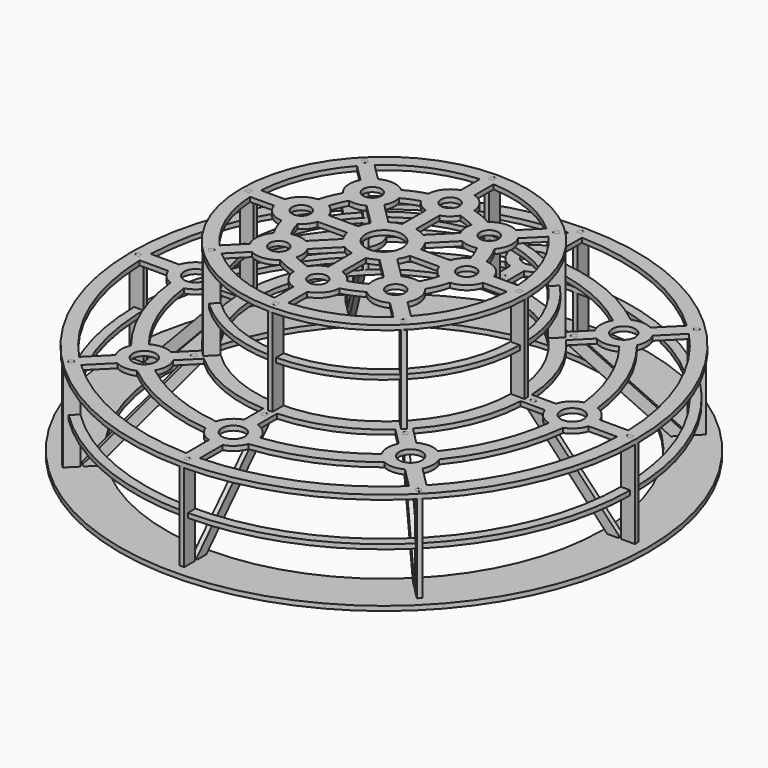
from build123d import *

# Parameters (mm, degrees)
F4_R      = 550
F4_R_2    = 25
F4_R_3    = 280
F5_DEPTH  = 10
F6_R      = 310
F6_R_2    = 20
F6_R_3    = 40
F7_DEPTH  = 10
F8_R      = 575
F8_R_2    = 475
F9_DEPTH  = 10
F11_DEPTH = 5
F12_COUNT = 8
F13_R     = 520
F14_DEPTH = 10
F15_R     = 280
F16_DEPTH = 10
F17_COUNT = 8


with BuildPart() as f5:
    # F4 (on Top) → F5 (new body)
    with BuildSketch(Plane.XY):
        Circle(F4_R)
        Polygon((-374.0594872477, -375.4737008101), (-371.3017708011, -378.2314172567), (-378.3728386129, -385.3024850685), (-381.1305550595, -382.5447686219), (-382.5447686219, -382.5447686219), (-382.5447686219, -381.1305550595), (-385.3024850685, -378.3728386129), (-378.2314172567, -371.3017708011), (-375.4737008101, -374.0594872477), (-374.0594872477, -374.0594872477), align=None, mode=Mode.SUBTRACT)
        with Locations((-289.9137802865, -289.9137802865)):
            Circle(F4_R_2, mode=Mode.SUBTRACT)
        with BuildLine():
            ThreePointArc((-46.8602222393, -427.4390243902), (-34.4319247471, -446.2552418033), (-15, -457.6969600708))
            Line((-15, -457.6969600708), (-15, -519.783608822))
            ThreePointArc((-15, -519.783608822), (-198.9953848298, -480.4173569059), (-356.9359128298, -378.1491162654))
            Line((-356.9359128298, -378.1491162654), (-313.0340224768, -334.2472259124))
            ThreePointArc((-313.0340224768, -334.2472259124), (-291.2030601412, -339.8971550971), (-269.1098517768, -335.3802136034))
            ThreePointArc((-269.1098517768, -335.3802136034), (-164.553875917, -397.2681989799), (-46.8602222393, -427.4390243902))
        make_face(mode=Mode.SUBTRACT)
        with BuildLine():
            Line((-15, -309.6368841078), (-15, -362.3030399292))
            ThreePointArc((-15, -362.3030399292), (-36.1104599854, -375.4162656782), (-48.3000733443, -397.0731707317))
            ThreePointArc((-48.3000733443, -397.0731707317), (-153.073372946, -369.5518130045), (-246.619822258, -314.9264410452))
            ThreePointArc((-246.619822258, -314.9264410452), (-239.9254361013, -290.9933383562), (-245.5803346606, -266.7935380962))
            Line((-245.5803346606, -266.7935380962), (-208.3397387403, -229.5529421759))
            ThreePointArc((-208.3397387403, -229.5529421759), (-118.6318640332, -286.4026550785), (-15, -309.6368841078))
        make_face(mode=Mode.SUBTRACT)
        with BuildLine():
            Line((-519.783608822, -15), (-457.6969600708, -15))
            ThreePointArc((-457.6969600708, -15), (-446.2552418033, -34.4319247471), (-427.4390243902, -46.8602222393))
            ThreePointArc((-427.4390243902, -46.8602222393), (-397.2681989799, -164.553875917), (-335.3802136034, -269.1098517768))
            ThreePointArc((-335.3802136034, -269.1098517768), (-339.8971550971, -291.2030601412), (-334.2472259124, -313.0340224768))
            Line((-334.2472259124, -313.0340224768), (-378.1491162654, -356.9359128298))
            ThreePointArc((-378.1491162654, -356.9359128298), (-480.4173569059, -198.9953848298), (-519.783608822, -15))
        make_face(mode=Mode.SUBTRACT)
        with BuildLine():
            ThreePointArc((-397.0731707317, -48.3000733443), (-375.4162656782, -36.1104599854), (-362.3030399292, -15))
            Line((-362.3030399292, -15), (-309.6368841078, -15))
            ThreePointArc((-309.6368841078, -15), (-286.4026550785, -118.6318640332), (-229.5529421759, -208.3397387403))
            Line((-229.5529421759, -208.3397387403), (-266.7935380962, -245.5803346606))
            ThreePointArc((-266.7935380962, -245.5803346606), (-290.9933383562, -239.9254361013), (-314.9264410452, -246.619822258))
            ThreePointArc((-314.9264410452, -246.619822258), (-369.5518130045, -153.073372946), (-397.0731707317, -48.3000733443))
        make_face(mode=Mode.SUBTRACT)
        Polygon((-236.8100610194, -229.8804145637), (-229.7389932075, -222.8093467519), (-226.9812767609, -225.5670631985), (-225.5670631985, -225.5670631985), (-225.5670631985, -226.9812767609), (-222.8093467519, -229.7389932075), (-229.8804145637, -236.8100610194), (-232.6381310104, -234.0523445727), (-234.0523445727, -234.0523445727), (-234.0523445727, -232.6381310104), align=None, mode=Mode.SUBTRACT)
        Polygon((-215.5968575838, -208.6672111282), (-208.5257897719, -201.5961433163), (-205.7680733253, -204.3538597629), (-204.3538597629, -204.3538597629), (-204.3538597629, -205.7680733253), (-201.5961433163, -208.5257897719), (-208.6672111282, -215.5968575838), (-211.4249275748, -212.8391411372), (-212.8391411372, -212.8391411372), (-212.8391411372, -211.4249275748), align=None, mode=Mode.SUBTRACT)
        Polygon((1, -530), (4.9, -530), (4.9, -540), (1, -540), (0, -541), (-1, -540), (-4.9, -540), (-4.9, -530), (-1, -530), (0, -529), align=None, mode=Mode.SUBTRACT)
        with BuildLine():
            ThreePointArc((356.9359128298, -378.1491162654), (198.9953848298, -480.4173569059), (15, -519.783608822))
            Line((15, -519.783608822), (15, -457.6969600708))
            ThreePointArc((15, -457.6969600708), (34.4319247471, -446.2552418033), (46.8602222393, -427.4390243902))
            ThreePointArc((46.8602222393, -427.4390243902), (164.553875917, -397.2681989799), (269.1098517768, -335.3802136034))
            ThreePointArc((269.1098517768, -335.3802136034), (291.2030601412, -339.8971550971), (313.0340224768, -334.2472259124))
            Line((313.0340224768, -334.2472259124), (356.9359128298, -378.1491162654))
        make_face(mode=Mode.SUBTRACT)
        with Locations((0, -410)):
            Circle(F4_R_2, mode=Mode.SUBTRACT)
        Polygon((-4.9, -330), (-4.9, -320), (-1, -320), (0, -319), (1, -320), (4.9, -320), (4.9, -330), (1, -330), (0, -331), (-1, -330), align=None, mode=Mode.SUBTRACT)
        Polygon((-4.9, -300), (-4.9, -290), (-1, -290), (0, -289), (1, -290), (4.9, -290), (4.9, -300), (1, -300), (0, -301), (-1, -300), align=None, mode=Mode.SUBTRACT)
        with BuildLine():
            ThreePointArc((246.619822258, -314.9264410452), (153.073372946, -369.5518130045), (48.3000733443, -397.0731707317))
            ThreePointArc((48.3000733443, -397.0731707317), (36.1104599854, -375.4162656782), (15, -362.3030399292))
            Line((15, -362.3030399292), (15, -309.6368841078))
            ThreePointArc((15, -309.6368841078), (118.6318640332, -286.4026550785), (208.3397387403, -229.5529421759))
            Line((208.3397387403, -229.5529421759), (245.5803346606, -266.7935380962))
            ThreePointArc((245.5803346606, -266.7935380962), (239.9254361013, -290.9933383562), (246.619822258, -314.9264410452))
        make_face(mode=Mode.SUBTRACT)
        Polygon((375.4737008101, -374.0594872477), (378.2314172567, -371.3017708011), (385.3024850685, -378.3728386129), (382.5447686219, -381.1305550595), (382.5447686219, -382.5447686219), (381.1305550595, -382.5447686219), (378.3728386129, -385.3024850685), (371.3017708011, -378.2314172567), (374.0594872477, -375.4737008101), (374.0594872477, -374.0594872477), align=None, mode=Mode.SUBTRACT)
        with Locations((289.9137802865, -289.9137802865)):
            Circle(F4_R_2, mode=Mode.SUBTRACT)
        Polygon((229.8804145637, -236.8100610194), (222.8093467519, -229.7389932075), (225.5670631985, -226.9812767609), (225.5670631985, -225.5670631985), (226.9812767609, -225.5670631985), (229.7389932075, -222.8093467519), (236.8100610194, -229.8804145637), (234.0523445727, -232.6381310104), (234.0523445727, -234.0523445727), (232.6381310104, -234.0523445727), align=None, mode=Mode.SUBTRACT)
        Polygon((208.6672111282, -215.5968575838), (201.5961433163, -208.5257897719), (204.3538597629, -205.7680733253), (204.3538597629, -204.3538597629), (205.7680733253, -204.3538597629), (208.5257897719, -201.5961433163), (215.5968575838, -208.6672111282), (212.8391411372, -211.4249275748), (212.8391411372, -212.8391411372), (211.4249275748, -212.8391411372), align=None, mode=Mode.SUBTRACT)
        with BuildLine():
            Line((378.1491162654, -356.9359128298), (334.2472259124, -313.0340224768))
            ThreePointArc((334.2472259124, -313.0340224768), (339.8971550971, -291.2030601412), (335.3802136034, -269.1098517768))
            ThreePointArc((335.3802136034, -269.1098517768), (397.2681989799, -164.553875917), (427.4390243902, -46.8602222393))
            ThreePointArc((427.4390243902, -46.8602222393), (446.2552418033, -34.4319247471), (457.6969600708, -15))
            Line((457.6969600708, -15), (519.783608822, -15))
            ThreePointArc((519.783608822, -15), (480.4173569059, -198.9953848298), (378.1491162654, -356.9359128298))
        make_face(mode=Mode.SUBTRACT)
        with BuildLine():
            ThreePointArc((314.9264410452, -246.619822258), (290.9933383562, -239.9254361013), (266.7935380962, -245.5803346606))
            Line((266.7935380962, -245.5803346606), (229.5529421759, -208.3397387403))
            ThreePointArc((229.5529421759, -208.3397387403), (286.4026550785, -118.6318640332), (309.6368841078, -15))
            Line((309.6368841078, -15), (362.3030399292, -15))
            ThreePointArc((362.3030399292, -15), (375.4162656782, -36.1104599854), (397.0731707317, -48.3000733443))
            ThreePointArc((397.0731707317, -48.3000733443), (369.5518130045, -153.073372946), (314.9264410452, -246.619822258))
        make_face(mode=Mode.SUBTRACT)
        Polygon((-530, -1), (-530, -4.9), (-540, -4.9), (-540, -1), (-541, 0), (-540, 1), (-540, 4.9), (-530, 4.9), (-530, 1), (-529, 0), align=None, mode=Mode.SUBTRACT)
        with Locations((-410, 0)):
            Circle(F4_R_2, mode=Mode.SUBTRACT)
        Polygon((-330, 4.9), (-320, 4.9), (-320, 1), (-319, 0), (-320, -1), (-320, -4.9), (-330, -4.9), (-330, -1), (-331, 0), (-330, 1), align=None, mode=Mode.SUBTRACT)
        Polygon((-300, 4.9), (-290, 4.9), (-290, 1), (-289, 0), (-290, -1), (-290, -4.9), (-300, -4.9), (-300, -1), (-301, 0), (-300, 1), align=None, mode=Mode.SUBTRACT)
        with BuildLine():
            ThreePointArc((-314.9264410452, 246.619822258), (-290.9933383562, 239.9254361013), (-266.7935380962, 245.5803346606))
            Line((-266.7935380962, 245.5803346606), (-229.5529421759, 208.3397387403))
            ThreePointArc((-229.5529421759, 208.3397387403), (-286.4026550785, 118.6318640332), (-309.6368841078, 15))
            Line((-309.6368841078, 15), (-362.3030399292, 15))
            ThreePointArc((-362.3030399292, 15), (-375.4162656782, 36.1104599854), (-397.0731707317, 48.3000733443))
            ThreePointArc((-397.0731707317, 48.3000733443), (-369.5518130045, 153.073372946), (-314.9264410452, 246.619822258))
        make_face(mode=Mode.SUBTRACT)
        with BuildLine():
            Line((-378.1491162654, 356.9359128298), (-334.2472259124, 313.0340224768))
            ThreePointArc((-334.2472259124, 313.0340224768), (-339.8971550971, 291.2030601412), (-335.3802136034, 269.1098517768))
            ThreePointArc((-335.3802136034, 269.1098517768), (-397.2681989799, 164.553875917), (-427.4390243902, 46.8602222393))
            ThreePointArc((-427.4390243902, 46.8602222393), (-446.2552418033, 34.4319247471), (-457.6969600708, 15))
            Line((-457.6969600708, 15), (-519.783608822, 15))
            ThreePointArc((-519.783608822, 15), (-480.4173569059, 198.9953848298), (-378.1491162654, 356.9359128298))
        make_face(mode=Mode.SUBTRACT)
        Polygon((-208.6672111282, 215.5968575838), (-201.5961433163, 208.5257897719), (-204.3538597629, 205.7680733253), (-204.3538597629, 204.3538597629), (-205.7680733253, 204.3538597629), (-208.5257897719, 201.5961433163), (-215.5968575838, 208.6672111282), (-212.8391411372, 211.4249275748), (-212.8391411372, 212.8391411372), (-211.4249275748, 212.8391411372), align=None, mode=Mode.SUBTRACT)
        Polygon((-229.8804145637, 236.8100610194), (-222.8093467519, 229.7389932075), (-225.5670631985, 226.9812767609), (-225.5670631985, 225.5670631985), (-226.9812767609, 225.5670631985), (-229.7389932075, 222.8093467519), (-236.8100610194, 229.8804145637), (-234.0523445727, 232.6381310104), (-234.0523445727, 234.0523445727), (-232.6381310104, 234.0523445727), align=None, mode=Mode.SUBTRACT)
        with Locations((-289.9137802865, 289.9137802865)):
            Circle(F4_R_2, mode=Mode.SUBTRACT)
        Polygon((-375.4737008101, 374.0594872477), (-378.2314172567, 371.3017708011), (-385.3024850685, 378.3728386129), (-382.5447686219, 381.1305550595), (-382.5447686219, 382.5447686219), (-381.1305550595, 382.5447686219), (-378.3728386129, 385.3024850685), (-371.3017708011, 378.2314172567), (-374.0594872477, 375.4737008101), (-374.0594872477, 374.0594872477), align=None, mode=Mode.SUBTRACT)
        with BuildLine():
            ThreePointArc((-48.3000733443, 397.0731707317), (-36.1104599854, 375.4162656782), (-15, 362.3030399292))
            Line((-15, 362.3030399292), (-15, 309.6368841078))
            ThreePointArc((-15, 309.6368841078), (-118.6318640332, 286.4026550785), (-208.3397387403, 229.5529421759))
            Line((-208.3397387403, 229.5529421759), (-245.5803346606, 266.7935380962))
            ThreePointArc((-245.5803346606, 266.7935380962), (-239.9254361013, 290.9933383562), (-246.619822258, 314.9264410452))
            ThreePointArc((-246.619822258, 314.9264410452), (-153.073372946, 369.5518130045), (-48.3000733443, 397.0731707317))
        make_face(mode=Mode.SUBTRACT)
        with BuildLine():
            Line((-15, 519.783608822), (-15, 457.6969600708))
            ThreePointArc((-15, 457.6969600708), (-34.4319247471, 446.2552418033), (-46.8602222393, 427.4390243902))
            ThreePointArc((-46.8602222393, 427.4390243902), (-164.553875917, 397.2681989799), (-269.1098517768, 335.3802136034))
            ThreePointArc((-269.1098517768, 335.3802136034), (-291.2030601412, 339.8971550971), (-313.0340224768, 334.2472259124))
            Line((-313.0340224768, 334.2472259124), (-356.9359128298, 378.1491162654))
            ThreePointArc((-356.9359128298, 378.1491162654), (-198.9953848298, 480.4173569059), (-15, 519.783608822))
        make_face(mode=Mode.SUBTRACT)
        Circle(F4_R_3, mode=Mode.SUBTRACT)
        Polygon((215.5968575838, 208.6672111282), (208.5257897719, 201.5961433163), (205.7680733253, 204.3538597629), (204.3538597629, 204.3538597629), (204.3538597629, 205.7680733253), (201.5961433163, 208.5257897719), (208.6672111282, 215.5968575838), (211.4249275748, 212.8391411372), (212.8391411372, 212.8391411372), (212.8391411372, 211.4249275748), align=None, mode=Mode.SUBTRACT)
        Polygon((236.8100610194, 229.8804145637), (229.7389932075, 222.8093467519), (226.9812767609, 225.5670631985), (225.5670631985, 225.5670631985), (225.5670631985, 226.9812767609), (222.8093467519, 229.7389932075), (229.8804145637, 236.8100610194), (232.6381310104, 234.0523445727), (234.0523445727, 234.0523445727), (234.0523445727, 232.6381310104), align=None, mode=Mode.SUBTRACT)
        Polygon((300, -4.9), (290, -4.9), (290, -1), (289, 0), (290, 1), (290, 4.9), (300, 4.9), (300, 1), (301, 0), (300, -1), align=None, mode=Mode.SUBTRACT)
        Polygon((330, -4.9), (320, -4.9), (320, -1), (319, 0), (320, 1), (320, 4.9), (330, 4.9), (330, 1), (331, 0), (330, -1), align=None, mode=Mode.SUBTRACT)
        with Locations((410, 0)):
            Circle(F4_R_2, mode=Mode.SUBTRACT)
        with BuildLine():
            ThreePointArc((397.0731707317, 48.3000733443), (375.4162656782, 36.1104599854), (362.3030399292, 15))
            Line((362.3030399292, 15), (309.6368841078, 15))
            ThreePointArc((309.6368841078, 15), (286.4026550785, 118.6318640332), (229.5529421759, 208.3397387403))
            Line((229.5529421759, 208.3397387403), (266.7935380962, 245.5803346606))
            ThreePointArc((266.7935380962, 245.5803346606), (290.9933383562, 239.9254361013), (314.9264410452, 246.619822258))
            ThreePointArc((314.9264410452, 246.619822258), (369.5518130045, 153.073372946), (397.0731707317, 48.3000733443))
        make_face(mode=Mode.SUBTRACT)
        Polygon((530, 1), (530, 4.9), (540, 4.9), (540, 1), (541, 0), (540, -1), (540, -4.9), (530, -4.9), (530, -1), (529, 0), align=None, mode=Mode.SUBTRACT)
        with BuildLine():
            Line((519.783608822, 15), (457.6969600708, 15))
            ThreePointArc((457.6969600708, 15), (446.2552418033, 34.4319247471), (427.4390243902, 46.8602222393))
            ThreePointArc((427.4390243902, 46.8602222393), (397.2681989799, 164.553875917), (335.3802136034, 269.1098517768))
            ThreePointArc((335.3802136034, 269.1098517768), (339.8971550971, 291.2030601412), (334.2472259124, 313.0340224768))
            Line((334.2472259124, 313.0340224768), (378.1491162654, 356.9359128298))
            ThreePointArc((378.1491162654, 356.9359128298), (480.4173569059, 198.9953848298), (519.783608822, 15))
        make_face(mode=Mode.SUBTRACT)
        Polygon((4.9, 300), (4.9, 290), (1, 290), (0, 289), (-1, 290), (-4.9, 290), (-4.9, 300), (-1, 300), (0, 301), (1, 300), align=None, mode=Mode.SUBTRACT)
        Polygon((4.9, 330), (4.9, 320), (1, 320), (0, 319), (-1, 320), (-4.9, 320), (-4.9, 330), (-1, 330), (0, 331), (1, 330), align=None, mode=Mode.SUBTRACT)
        with BuildLine():
            ThreePointArc((246.619822258, 314.9264410452), (239.9254361013, 290.9933383562), (245.5803346606, 266.7935380962))
            Line((245.5803346606, 266.7935380962), (208.3397387403, 229.5529421759))
            ThreePointArc((208.3397387403, 229.5529421759), (118.6318640332, 286.4026550785), (15, 309.6368841078))
            Line((15, 309.6368841078), (15, 362.3030399292))
            ThreePointArc((15, 362.3030399292), (36.1104599854, 375.4162656782), (48.3000733443, 397.0731707317))
            ThreePointArc((48.3000733443, 397.0731707317), (153.073372946, 369.5518130045), (246.619822258, 314.9264410452))
        make_face(mode=Mode.SUBTRACT)
        with Locations((0, 410)):
            Circle(F4_R_2, mode=Mode.SUBTRACT)
        Polygon((4.9, 540), (4.9, 530), (1, 530), (0, 529), (-1, 530), (-4.9, 530), (-4.9, 540), (-1, 540), (0, 541), (1, 540), align=None, mode=Mode.SUBTRACT)
        with BuildLine():
            Line((356.9359128298, 378.1491162654), (313.0340224768, 334.2472259124))
            ThreePointArc((313.0340224768, 334.2472259124), (291.2030601412, 339.8971550971), (269.1098517768, 335.3802136034))
            ThreePointArc((269.1098517768, 335.3802136034), (164.553875917, 397.2681989799), (46.8602222393, 427.4390243902))
            ThreePointArc((46.8602222393, 427.4390243902), (34.4319247471, 446.2552418033), (15, 457.6969600708))
            Line((15, 457.6969600708), (15, 519.783608822))
            ThreePointArc((15, 519.783608822), (198.9953848298, 480.4173569059), (356.9359128298, 378.1491162654))
        make_face(mode=Mode.SUBTRACT)
        with Locations((289.9137802865, 289.9137802865)):
            Circle(F4_R_2, mode=Mode.SUBTRACT)
        Polygon((374.0594872477, 375.4737008101), (371.3017708011, 378.2314172567), (378.3728386129, 385.3024850685), (381.1305550595, 382.5447686219), (382.5447686219, 382.5447686219), (382.5447686219, 381.1305550595), (385.3024850685, 378.3728386129), (378.2314172567, 371.3017708011), (375.4737008101, 374.0594872477), (374.0594872477, 374.0594872477), align=None, mode=Mode.SUBTRACT)
    extrude(amount=F5_DEPTH)


with BuildPart() as f7:
    # F6 (on offset) → F7 (new body)
    with BuildSketch(Plane.XY.offset(200)):
        Circle(F6_R)
        Polygon((-204.3538597629, -204.3538597629), (-204.3538597629, -205.7680733253), (-201.5961433163, -208.5257897719), (-208.6672111282, -215.5968575838), (-211.4249275748, -212.8391411372), (-212.8391411372, -212.8391411372), (-212.8391411372, -211.4249275748), (-215.5968575838, -208.6672111282), (-208.5257897719, -201.5961433163), (-205.7680733253, -204.3538597629), align=None, mode=Mode.SUBTRACT)
        with BuildLine():
            ThreePointArc((-49.888765157, -183.3333333333), (-39.3023002536, -210.9084000682), (-15, -227.6969600708))
            Line((-15, -227.6969600708), (-15, -279.5979256003))
            ThreePointArc((-15, -279.5979256003), (-107.1513610622, -258.6862691032), (-187.0989874799, -208.3121909155))
            Line((-187.0989874799, -208.3121909155), (-150.3994628039, -171.6126662395))
            ThreePointArc((-150.3994628039, -171.6126662395), (-121.3438368718, -176.925682923), (-94.35955907, -164.9129273651))
            ThreePointArc((-94.35955907, -164.9129273651), (-72.7098521494, -175.5371111771), (-49.888765157, -183.3333333333))
        make_face(mode=Mode.SUBTRACT)
        with BuildLine():
            Line((-279.5979256003, -15), (-227.6969600708, -15))
            ThreePointArc((-227.6969600708, -15), (-210.9084000682, -39.3023002536), (-183.3333333333, -49.888765157))
            ThreePointArc((-183.3333333333, -49.888765157), (-175.5371111771, -72.7098521494), (-164.9129273651, -94.35955907))
            ThreePointArc((-164.9129273651, -94.35955907), (-176.925682923, -121.3438368718), (-171.6126662395, -150.3994628039))
            Line((-171.6126662395, -150.3994628039), (-208.3121909155, -187.0989874799))
            ThreePointArc((-208.3121909155, -187.0989874799), (-258.6862691032, -107.1513610622), (-279.5979256003, -15))
        make_face(mode=Mode.SUBTRACT)
        with Locations((-127.2792206136, -127.2792206136)):
            Circle(F6_R_2, mode=Mode.SUBTRACT)
        with BuildLine():
            Line((-15, -68.3739716559), (-15, -132.3030399292))
            ThreePointArc((-15, -132.3030399292), (-30.9028195191, -140.6933116916), (-42.8093317968, -154.1666666667))
            ThreePointArc((-42.8093317968, -154.1666666667), (-61.2293491784, -147.8207252018), (-78.7415266213, -139.2830642445))
            ThreePointArc((-78.7415266213, -139.2830642445), (-77.633601525, -121.3367880044), (-82.9457749877, -104.1589784233))
            Line((-82.9457749877, -104.1589784233), (-37.7410972967, -58.9543007323))
            ThreePointArc((-37.7410972967, -58.9543007323), (-26.7878402656, -64.6715672758), (-15, -68.3739716559))
        make_face(mode=Mode.SUBTRACT)
        with BuildLine():
            Line((-132.3030399292, -15), (-68.3739716559, -15))
            ThreePointArc((-68.3739716559, -15), (-64.6715672758, -26.7878402656), (-58.9543007323, -37.7410972967))
            Line((-58.9543007323, -37.7410972967), (-104.1589784233, -82.9457749877))
            ThreePointArc((-104.1589784233, -82.9457749877), (-121.3367880044, -77.633601525), (-139.2830642445, -78.7415266213))
            ThreePointArc((-139.2830642445, -78.7415266213), (-147.8207252018, -61.2293491784), (-154.1666666667, -42.8093317968))
            ThreePointArc((-154.1666666667, -42.8093317968), (-140.6933116916, -30.9028195191), (-132.3030399292, -15))
        make_face(mode=Mode.SUBTRACT)
        Polygon((0, -289), (1, -290), (4.9, -290), (4.9, -300), (1, -300), (0, -301), (-1, -300), (-4.9, -300), (-4.9, -290), (-1, -290), align=None, mode=Mode.SUBTRACT)
        with Locations((0, -180)):
            Circle(F6_R_2, mode=Mode.SUBTRACT)
        with BuildLine():
            ThreePointArc((15, -227.6969600708), (39.3023002536, -210.9084000682), (49.888765157, -183.3333333333))
            ThreePointArc((49.888765157, -183.3333333333), (72.7098521494, -175.5371111771), (94.35955907, -164.9129273651))
            ThreePointArc((94.35955907, -164.9129273651), (121.3438368718, -176.925682923), (150.3994628039, -171.6126662395))
            Line((150.3994628039, -171.6126662395), (187.0989874799, -208.3121909155))
            ThreePointArc((187.0989874799, -208.3121909155), (107.1513610622, -258.6862691032), (15, -279.5979256003))
            Line((15, -279.5979256003), (15, -227.6969600708))
        make_face(mode=Mode.SUBTRACT)
        Polygon((204.3538597629, -204.3538597629), (205.7680733253, -204.3538597629), (208.5257897719, -201.5961433163), (215.5968575838, -208.6672111282), (212.8391411372, -211.4249275748), (212.8391411372, -212.8391411372), (211.4249275748, -212.8391411372), (208.6672111282, -215.5968575838), (201.5961433163, -208.5257897719), (204.3538597629, -205.7680733253), align=None, mode=Mode.SUBTRACT)
        with BuildLine():
            ThreePointArc((78.7415266213, -139.2830642445), (61.2293491784, -147.8207252018), (42.8093317968, -154.1666666667))
            ThreePointArc((42.8093317968, -154.1666666667), (30.9028195191, -140.6933116916), (15, -132.3030399292))
            Line((15, -132.3030399292), (15, -68.3739716559))
            ThreePointArc((15, -68.3739716559), (26.7878402656, -64.6715672758), (37.7410972967, -58.9543007323))
            Line((37.7410972967, -58.9543007323), (82.9457749877, -104.1589784233))
            ThreePointArc((82.9457749877, -104.1589784233), (77.633601525, -121.3367880044), (78.7415266213, -139.2830642445))
        make_face(mode=Mode.SUBTRACT)
        with Locations((127.2792206136, -127.2792206136)):
            Circle(F6_R_2, mode=Mode.SUBTRACT)
        with BuildLine():
            Line((104.1589784233, -82.9457749877), (58.9543007323, -37.7410972967))
            ThreePointArc((58.9543007323, -37.7410972967), (64.6715672758, -26.7878402656), (68.3739716559, -15))
            Line((68.3739716559, -15), (132.3030399292, -15))
            ThreePointArc((132.3030399292, -15), (140.6933116916, -30.9028195191), (154.1666666667, -42.8093317968))
            ThreePointArc((154.1666666667, -42.8093317968), (147.8207252018, -61.2293491784), (139.2830642445, -78.7415266213))
            ThreePointArc((139.2830642445, -78.7415266213), (121.3367880044, -77.633601525), (104.1589784233, -82.9457749877))
        make_face(mode=Mode.SUBTRACT)
        with BuildLine():
            Line((208.3121909155, -187.0989874799), (171.6126662395, -150.3994628039))
            ThreePointArc((171.6126662395, -150.3994628039), (176.925682923, -121.3438368718), (164.9129273651, -94.35955907))
            ThreePointArc((164.9129273651, -94.35955907), (175.5371111771, -72.7098521494), (183.3333333333, -49.888765157))
            ThreePointArc((183.3333333333, -49.888765157), (210.9084000682, -39.3023002536), (227.6969600708, -15))
            Line((227.6969600708, -15), (279.5979256003, -15))
            ThreePointArc((279.5979256003, -15), (258.6862691032, -107.1513610622), (208.3121909155, -187.0989874799))
        make_face(mode=Mode.SUBTRACT)
        Polygon((-289, 0), (-290, -1), (-290, -4.9), (-300, -4.9), (-300, -1), (-301, 0), (-300, 1), (-300, 4.9), (-290, 4.9), (-290, 1), align=None, mode=Mode.SUBTRACT)
        with Locations((-180, 0)):
            Circle(F6_R_2, mode=Mode.SUBTRACT)
        with BuildLine():
            Line((-208.3121909155, 187.0989874799), (-171.6126662395, 150.3994628039))
            ThreePointArc((-171.6126662395, 150.3994628039), (-176.925682923, 121.3438368718), (-164.9129273651, 94.35955907))
            ThreePointArc((-164.9129273651, 94.35955907), (-175.5371111771, 72.7098521494), (-183.3333333333, 49.888765157))
            ThreePointArc((-183.3333333333, 49.888765157), (-210.9084000682, 39.3023002536), (-227.6969600708, 15))
            Line((-227.6969600708, 15), (-279.5979256003, 15))
            ThreePointArc((-279.5979256003, 15), (-258.6862691032, 107.1513610622), (-208.3121909155, 187.0989874799))
        make_face(mode=Mode.SUBTRACT)
        with BuildLine():
            Line((-104.1589784233, 82.9457749877), (-58.9543007323, 37.7410972967))
            ThreePointArc((-58.9543007323, 37.7410972967), (-64.6715672758, 26.7878402656), (-68.3739716559, 15))
            Line((-68.3739716559, 15), (-132.3030399292, 15))
            ThreePointArc((-132.3030399292, 15), (-140.6933116916, 30.9028195191), (-154.1666666667, 42.8093317968))
            ThreePointArc((-154.1666666667, 42.8093317968), (-147.8207252018, 61.2293491784), (-139.2830642445, 78.7415266213))
            ThreePointArc((-139.2830642445, 78.7415266213), (-121.3367880044, 77.633601525), (-104.1589784233, 82.9457749877))
        make_face(mode=Mode.SUBTRACT)
        with Locations((-127.2792206136, 127.2792206136)):
            Circle(F6_R_2, mode=Mode.SUBTRACT)
        with BuildLine():
            Line((-15, 132.3030399292), (-15, 68.3739716559))
            ThreePointArc((-15, 68.3739716559), (-26.7878402656, 64.6715672758), (-37.7410972967, 58.9543007323))
            Line((-37.7410972967, 58.9543007323), (-82.9457749877, 104.1589784233))
            ThreePointArc((-82.9457749877, 104.1589784233), (-77.633601525, 121.3367880044), (-78.7415266213, 139.2830642445))
            ThreePointArc((-78.7415266213, 139.2830642445), (-61.2293491784, 147.8207252018), (-42.8093317968, 154.1666666667))
            ThreePointArc((-42.8093317968, 154.1666666667), (-30.9028195191, 140.6933116916), (-15, 132.3030399292))
        make_face(mode=Mode.SUBTRACT)
        Polygon((-204.3538597629, 204.3538597629), (-205.7680733253, 204.3538597629), (-208.5257897719, 201.5961433163), (-215.5968575838, 208.6672111282), (-212.8391411372, 211.4249275748), (-212.8391411372, 212.8391411372), (-211.4249275748, 212.8391411372), (-208.6672111282, 215.5968575838), (-201.5961433163, 208.5257897719), (-204.3538597629, 205.7680733253), align=None, mode=Mode.SUBTRACT)
        with BuildLine():
            Line((-15, 279.5979256003), (-15, 227.6969600708))
            ThreePointArc((-15, 227.6969600708), (-39.3023002536, 210.9084000682), (-49.888765157, 183.3333333333))
            ThreePointArc((-49.888765157, 183.3333333333), (-72.7098521494, 175.5371111771), (-94.35955907, 164.9129273651))
            ThreePointArc((-94.35955907, 164.9129273651), (-121.3438368718, 176.925682923), (-150.3994628039, 171.6126662395))
            Line((-150.3994628039, 171.6126662395), (-187.0989874799, 208.3121909155))
            ThreePointArc((-187.0989874799, 208.3121909155), (-107.1513610622, 258.6862691032), (-15, 279.5979256003))
        make_face(mode=Mode.SUBTRACT)
        Circle(F6_R_3, mode=Mode.SUBTRACT)
        with BuildLine():
            Line((132.3030399292, 15), (68.3739716559, 15))
            ThreePointArc((68.3739716559, 15), (64.6715672758, 26.7878402656), (58.9543007323, 37.7410972967))
            Line((58.9543007323, 37.7410972967), (104.1589784233, 82.9457749877))
            ThreePointArc((104.1589784233, 82.9457749877), (121.3367880044, 77.633601525), (139.2830642445, 78.7415266213))
            ThreePointArc((139.2830642445, 78.7415266213), (147.8207252018, 61.2293491784), (154.1666666667, 42.8093317968))
            ThreePointArc((154.1666666667, 42.8093317968), (140.6933116916, 30.9028195191), (132.3030399292, 15))
        make_face(mode=Mode.SUBTRACT)
        with BuildLine():
            Line((82.9457749877, 104.1589784233), (37.7410972967, 58.9543007323))
            ThreePointArc((37.7410972967, 58.9543007323), (26.7878402656, 64.6715672758), (15, 68.3739716559))
            Line((15, 68.3739716559), (15, 132.3030399292))
            ThreePointArc((15, 132.3030399292), (30.9028195191, 140.6933116916), (42.8093317968, 154.1666666667))
            ThreePointArc((42.8093317968, 154.1666666667), (61.2293491784, 147.8207252018), (78.7415266213, 139.2830642445))
            ThreePointArc((78.7415266213, 139.2830642445), (77.633601525, 121.3367880044), (82.9457749877, 104.1589784233))
        make_face(mode=Mode.SUBTRACT)
        with Locations((127.2792206136, 127.2792206136)):
            Circle(F6_R_2, mode=Mode.SUBTRACT)
        with Locations((180, 0)):
            Circle(F6_R_2, mode=Mode.SUBTRACT)
        Polygon((289, 0), (290, 1), (290, 4.9), (300, 4.9), (300, 1), (301, 0), (300, -1), (300, -4.9), (290, -4.9), (290, -1), align=None, mode=Mode.SUBTRACT)
        with BuildLine():
            Line((279.5979256003, 15), (227.6969600708, 15))
            ThreePointArc((227.6969600708, 15), (210.9084000682, 39.3023002536), (183.3333333333, 49.888765157))
            ThreePointArc((183.3333333333, 49.888765157), (175.5371111771, 72.7098521494), (164.9129273651, 94.35955907))
            ThreePointArc((164.9129273651, 94.35955907), (176.925682923, 121.3438368718), (171.6126662395, 150.3994628039))
            Line((171.6126662395, 150.3994628039), (208.3121909155, 187.0989874799))
            ThreePointArc((208.3121909155, 187.0989874799), (258.6862691032, 107.1513610622), (279.5979256003, 15))
        make_face(mode=Mode.SUBTRACT)
        with Locations((0, 180)):
            Circle(F6_R_2, mode=Mode.SUBTRACT)
        with BuildLine():
            Line((187.0989874799, 208.3121909155), (150.3994628039, 171.6126662395))
            ThreePointArc((150.3994628039, 171.6126662395), (121.3438368718, 176.925682923), (94.35955907, 164.9129273651))
            ThreePointArc((94.35955907, 164.9129273651), (72.7098521494, 175.5371111771), (49.888765157, 183.3333333333))
            ThreePointArc((49.888765157, 183.3333333333), (39.3023002536, 210.9084000682), (15, 227.6969600708))
            Line((15, 227.6969600708), (15, 279.5979256003))
            ThreePointArc((15, 279.5979256003), (107.1513610622, 258.6862691032), (187.0989874799, 208.3121909155))
        make_face(mode=Mode.SUBTRACT)
        Polygon((-1, 290), (-4.9, 290), (-4.9, 300), (-1, 300), (0, 301), (1, 300), (4.9, 300), (4.9, 290), (1, 290), (0, 289), align=None, mode=Mode.SUBTRACT)
        Polygon((204.3538597629, 204.3538597629), (204.3538597629, 205.7680733253), (201.5961433163, 208.5257897719), (208.6672111282, 215.5968575838), (211.4249275748, 212.8391411372), (212.8391411372, 212.8391411372), (212.8391411372, 211.4249275748), (215.5968575838, 208.6672111282), (208.5257897719, 201.5961433163), (205.7680733253, 204.3538597629), align=None, mode=Mode.SUBTRACT)
    extrude(amount=F7_DEPTH)


with BuildPart() as f9:
    # F8 (on offset) → F9 (new body)
    with BuildSketch(Plane.XY.offset(-200)):
        Circle(F8_R)
        Polygon((-374.0594872477, -375.4737008101), (-371.3017708011, -378.2314172567), (-378.3728386129, -385.3024850685), (-381.1305550595, -382.5447686219), (-382.5447686219, -382.5447686219), (-382.5447686219, -381.1305550595), (-385.3024850685, -378.3728386129), (-378.2314172567, -371.3017708011), (-375.4737008101, -374.0594872477), (-374.0594872477, -374.0594872477), align=None, mode=Mode.SUBTRACT)
        Polygon((-364.089281633, -357.1596351773), (-357.0182138211, -350.0885673655), (-354.2604973745, -352.8462838121), (-352.8462838121, -352.8462838121), (-352.8462838121, -354.2604973745), (-350.0885673655, -357.0182138211), (-357.1596351773, -364.089281633), (-359.917351624, -361.3315651863), (-361.3315651863, -361.3315651863), (-361.3315651863, -359.917351624), align=None, mode=Mode.SUBTRACT)
        Polygon((1, -530), (4.9, -530), (4.9, -540), (1, -540), (0, -541), (-1, -540), (-4.9, -540), (-4.9, -530), (-1, -530), (0, -529), align=None, mode=Mode.SUBTRACT)
        Polygon((-4.9, -510), (-4.9, -500), (-1, -500), (0, -499), (1, -500), (4.9, -500), (4.9, -510), (1, -510), (0, -511), (-1, -510), align=None, mode=Mode.SUBTRACT)
        Polygon((375.4737008101, -374.0594872477), (378.2314172567, -371.3017708011), (385.3024850685, -378.3728386129), (382.5447686219, -381.1305550595), (382.5447686219, -382.5447686219), (381.1305550595, -382.5447686219), (378.3728386129, -385.3024850685), (371.3017708011, -378.2314172567), (374.0594872477, -375.4737008101), (374.0594872477, -374.0594872477), align=None, mode=Mode.SUBTRACT)
        Polygon((357.1596351773, -364.089281633), (350.0885673655, -357.0182138211), (352.8462838121, -354.2604973745), (352.8462838121, -352.8462838121), (354.2604973745, -352.8462838121), (357.0182138211, -350.0885673655), (364.089281633, -357.1596351773), (361.3315651863, -359.917351624), (361.3315651863, -361.3315651863), (359.917351624, -361.3315651863), align=None, mode=Mode.SUBTRACT)
        Polygon((-530, -1), (-530, -4.9), (-540, -4.9), (-540, -1), (-541, 0), (-540, 1), (-540, 4.9), (-530, 4.9), (-530, 1), (-529, 0), align=None, mode=Mode.SUBTRACT)
        Polygon((-510, 4.9), (-500, 4.9), (-500, 1), (-499, 0), (-500, -1), (-500, -4.9), (-510, -4.9), (-510, -1), (-511, 0), (-510, 1), align=None, mode=Mode.SUBTRACT)
        Polygon((-357.1596351773, 364.089281633), (-350.0885673655, 357.0182138211), (-352.8462838121, 354.2604973745), (-352.8462838121, 352.8462838121), (-354.2604973745, 352.8462838121), (-357.0182138211, 350.0885673655), (-364.089281633, 357.1596351773), (-361.3315651863, 359.917351624), (-361.3315651863, 361.3315651863), (-359.917351624, 361.3315651863), align=None, mode=Mode.SUBTRACT)
        Polygon((-375.4737008101, 374.0594872477), (-378.2314172567, 371.3017708011), (-385.3024850685, 378.3728386129), (-382.5447686219, 381.1305550595), (-382.5447686219, 382.5447686219), (-381.1305550595, 382.5447686219), (-378.3728386129, 385.3024850685), (-371.3017708011, 378.2314172567), (-374.0594872477, 375.4737008101), (-374.0594872477, 374.0594872477), align=None, mode=Mode.SUBTRACT)
        Circle(F8_R_2, mode=Mode.SUBTRACT)
        Polygon((510, -4.9), (500, -4.9), (500, -1), (499, 0), (500, 1), (500, 4.9), (510, 4.9), (510, 1), (511, 0), (510, -1), align=None, mode=Mode.SUBTRACT)
        Polygon((530, 1), (530, 4.9), (540, 4.9), (540, 1), (541, 0), (540, -1), (540, -4.9), (530, -4.9), (530, -1), (529, 0), align=None, mode=Mode.SUBTRACT)
        Polygon((4.9, 510), (4.9, 500), (1, 500), (0, 499), (-1, 500), (-4.9, 500), (-4.9, 510), (-1, 510), (0, 511), (1, 510), align=None, mode=Mode.SUBTRACT)
        Polygon((4.9, 540), (4.9, 530), (1, 530), (0, 529), (-1, 530), (-4.9, 530), (-4.9, 540), (-1, 540), (0, 541), (1, 540), align=None, mode=Mode.SUBTRACT)
        Polygon((364.089281633, 357.1596351773), (357.0182138211, 350.0885673655), (354.2604973745, 352.8462838121), (352.8462838121, 352.8462838121), (352.8462838121, 354.2604973745), (350.0885673655, 357.0182138211), (357.1596351773, 364.089281633), (359.917351624, 361.3315651863), (361.3315651863, 361.3315651863), (361.3315651863, 359.917351624), align=None, mode=Mode.SUBTRACT)
        Polygon((374.0594872477, 375.4737008101), (371.3017708011, 378.2314172567), (378.3728386129, 385.3024850685), (381.1305550595, 382.5447686219), (382.5447686219, 382.5447686219), (382.5447686219, 381.1305550595), (385.3024850685, 378.3728386129), (378.2314172567, 371.3017708011), (375.4737008101, 374.0594872477), (374.0594872477, 374.0594872477), align=None, mode=Mode.SUBTRACT)
    extrude(amount=F9_DEPTH)


with BuildPart() as f11:
    # F10 (on Right) → F11 (new body, symmetric)
    with BuildSketch(Plane.YZ):
        Polygon((550, 0), (540, 0), (540, 10), (530, 10), (530, 0), (520, 0), (520, -90.1), (530, -90.1), (530, -99.9), (520, -99.9), (520, -190), (530, -190), (530, -200), (540, -200), (540, -190), (550, -190), align=None)
    extrude(amount=F11_DEPTH, both=True)


with BuildPart() as f11b:
    # F10 (on Right) → F11, piece 2 (new body, symmetric)
    with BuildSketch(Plane.YZ):
        Polygon((290, 10), (290, 0), (300, 0), (300, 10), (310, 10), (310, 200), (300, 200), (300, 210), (290, 210), (290, 200), (280, 200), (280, 109.9), (290, 109.9), (290, 100.1), (280, 100.1), (280, 10), align=None)
    extrude(amount=F11_DEPTH, both=True)


with BuildPart() as f11c:
    # F10 (on Right) → F11, piece 3 (new body, symmetric)
    with BuildSketch(Plane.YZ):
        with BuildLine():
            Line((510, -190), (513.0253940016, -190))
            ThreePointArc((513.0253940016, -190), (515.7812697092, -188.1853898449), (515.2032520533, -184.9367660563))
            Line((515.2032520533, -184.9367660563), (340, 0))
            Line((340, 0), (330, 0))
            Line((330, 0), (330, 10))
            Line((330, 10), (320, 10))
            Line((320, 10), (320, 0))
            Line((320, 0), (310, 0))
            Line((310, 0), (490, -190))
            Line((490, -190), (500, -190))
            Line((500, -190), (500, -200))
            Line((500, -200), (510, -200))
            Line((510, -200), (510, -190))
        make_face()
    extrude(amount=F11_DEPTH, both=True)


with BuildPart() as f12_1:
    # F12: instance of F11
    add(f11.part.rotate(Axis((0, 0, 210), (0, 0, 1)), 1 * 360 / F12_COUNT))


with BuildPart() as f12_2:
    # F12: instance of F11
    add(f11.part.rotate(Axis((0, 0, 210), (0, 0, 1)), 2 * 360 / F12_COUNT))


with BuildPart() as f12_3:
    # F12: instance of F11
    add(f11.part.rotate(Axis((0, 0, 210), (0, 0, 1)), 3 * 360 / F12_COUNT))


with BuildPart() as f12_4:
    # F12: instance of F11
    add(f11.part.rotate(Axis((0, 0, 210), (0, 0, 1)), 4 * 360 / F12_COUNT))


with BuildPart() as f12_5:
    # F12: instance of F11
    add(f11.part.rotate(Axis((0, 0, 210), (0, 0, 1)), 5 * 360 / F12_COUNT))


with BuildPart() as f12_6:
    # F12: instance of F11
    add(f11.part.rotate(Axis((0, 0, 210), (0, 0, 1)), 6 * 360 / F12_COUNT))


with BuildPart() as f12_7:
    # F12: instance of F11
    add(f11.part.rotate(Axis((0, 0, 210), (0, 0, 1)), 7 * 360 / F12_COUNT))


with BuildPart() as f12_8:
    # F12: instance of F11b
    add(f11b.part.rotate(Axis((0, 0, 210), (0, 0, 1)), 1 * 360 / F12_COUNT))


with BuildPart() as f12_9:
    # F12: instance of F11b
    add(f11b.part.rotate(Axis((0, 0, 210), (0, 0, 1)), 2 * 360 / F12_COUNT))


with BuildPart() as f12_10:
    # F12: instance of F11b
    add(f11b.part.rotate(Axis((0, 0, 210), (0, 0, 1)), 3 * 360 / F12_COUNT))


with BuildPart() as f12_11:
    # F12: instance of F11b
    add(f11b.part.rotate(Axis((0, 0, 210), (0, 0, 1)), 4 * 360 / F12_COUNT))


with BuildPart() as f12_12:
    # F12: instance of F11b
    add(f11b.part.rotate(Axis((0, 0, 210), (0, 0, 1)), 5 * 360 / F12_COUNT))


with BuildPart() as f12_13:
    # F12: instance of F11b
    add(f11b.part.rotate(Axis((0, 0, 210), (0, 0, 1)), 6 * 360 / F12_COUNT))


with BuildPart() as f12_14:
    # F12: instance of F11b
    add(f11b.part.rotate(Axis((0, 0, 210), (0, 0, 1)), 7 * 360 / F12_COUNT))


with BuildPart() as f14:
    # F13 (on offset) → F14 (new body)
    with BuildSketch(Plane.XY.offset(-100)):
        with BuildLine():
            Line((-530, -5), (-539.9768513557, -5))
            ThreePointArc((-539.9768513557, -5), (-498.8949475561, -206.6490534771), (-385.3568271833, -378.2857593714))
            Line((-385.3568271833, -378.2857593714), (-378.3021279348, -371.2310601229))
            Line((-378.3021279348, -371.2310601229), (-371.2310601229, -378.3021279348))
            Line((-371.2310601229, -378.3021279348), (-378.2857593714, -385.3568271833))
            ThreePointArc((-378.2857593714, -385.3568271833), (-206.6490534771, -498.8949475561), (-5, -539.9768513557))
            Line((-5, -539.9768513557), (-5, -530))
            Line((-5, -530), (5, -530))
            Line((5, -530), (5, -539.9768513557))
            ThreePointArc((5, -539.9768513557), (206.6490534771, -498.8949475561), (378.2857593714, -385.3568271833))
            Line((378.2857593714, -385.3568271833), (371.2310601229, -378.3021279348))
            Line((371.2310601229, -378.3021279348), (378.3021279348, -371.2310601229))
            Line((378.3021279348, -371.2310601229), (385.3568271833, -378.2857593714))
            ThreePointArc((385.3568271833, -378.2857593714), (498.8949475561, -206.6490534771), (539.9768513557, -5))
            Line((539.9768513557, -5), (530, -5))
            Line((530, -5), (530, 5))
            Line((530, 5), (539.9768513557, 5))
            ThreePointArc((539.9768513557, 5), (498.8949475561, 206.6490534771), (385.3568271833, 378.2857593714))
            Line((385.3568271833, 378.2857593714), (378.3021279348, 371.2310601229))
            Line((378.3021279348, 371.2310601229), (371.2310601229, 378.3021279348))
            Line((371.2310601229, 378.3021279348), (378.2857593714, 385.3568271833))
            ThreePointArc((378.2857593714, 385.3568271833), (206.6490534771, 498.8949475561), (5, 539.9768513557))
            Line((5, 539.9768513557), (5, 530))
            Line((5, 530), (-5, 530))
            Line((-5, 530), (-5, 539.9768513557))
            ThreePointArc((-5, 539.9768513557), (-206.6490534771, 498.8949475561), (-378.2857593714, 385.3568271833))
            Line((-378.2857593714, 385.3568271833), (-371.2310601229, 378.3021279348))
            Line((-371.2310601229, 378.3021279348), (-378.3021279348, 371.2310601229))
            Line((-378.3021279348, 371.2310601229), (-385.3568271833, 378.2857593714))
            ThreePointArc((-385.3568271833, 378.2857593714), (-498.8949475561, 206.6490534771), (-539.9768513557, 5))
            Line((-539.9768513557, 5), (-530, 5))
            Line((-530, 5), (-530, -5))
        make_face()
        Circle(F13_R, mode=Mode.SUBTRACT)
    extrude(amount=F14_DEPTH)


with BuildPart() as f16:
    # F15 (on offset) → F16 (new body)
    with BuildSketch(Plane.XY.offset(100)):
        with BuildLine():
            Line((-290, -5), (-299.9583304394, -5))
            ThreePointArc((-299.9583304394, -5), (-277.1638597534, -114.8050297095), (-215.638103433, -208.5670356212))
            Line((-215.638103433, -208.5670356212), (-208.59650045, -201.5254326382))
            Line((-208.59650045, -201.5254326382), (-201.5254326382, -208.59650045))
            Line((-201.5254326382, -208.59650045), (-208.5670356212, -215.638103433))
            ThreePointArc((-208.5670356212, -215.638103433), (-114.8050297095, -277.1638597534), (-5, -299.9583304394))
            Line((-5, -299.9583304394), (-5, -290))
            Line((-5, -290), (5, -290))
            Line((5, -290), (5, -299.9583304394))
            ThreePointArc((5, -299.9583304394), (114.8050297095, -277.1638597534), (208.5670356212, -215.638103433))
            Line((208.5670356212, -215.638103433), (201.5254326382, -208.59650045))
            Line((201.5254326382, -208.59650045), (208.59650045, -201.5254326382))
            Line((208.59650045, -201.5254326382), (215.638103433, -208.5670356212))
            ThreePointArc((215.638103433, -208.5670356212), (277.1638597534, -114.8050297095), (299.9583304394, -5))
            Line((299.9583304394, -5), (290, -5))
            Line((290, -5), (290, 5))
            Line((290, 5), (299.9583304394, 5))
            ThreePointArc((299.9583304394, 5), (277.1638597534, 114.8050297095), (215.638103433, 208.5670356212))
            Line((215.638103433, 208.5670356212), (208.59650045, 201.5254326382))
            Line((208.59650045, 201.5254326382), (201.5254326382, 208.59650045))
            Line((201.5254326382, 208.59650045), (208.5670356212, 215.638103433))
            ThreePointArc((208.5670356212, 215.638103433), (114.8050297095, 277.1638597534), (5, 299.9583304394))
            Line((5, 299.9583304394), (5, 290))
            Line((5, 290), (-5, 290))
            Line((-5, 290), (-5, 299.9583304394))
            ThreePointArc((-5, 299.9583304394), (-114.8050297095, 277.1638597534), (-208.5670356212, 215.638103433))
            Line((-208.5670356212, 215.638103433), (-201.5254326382, 208.59650045))
            Line((-201.5254326382, 208.59650045), (-208.59650045, 201.5254326382))
            Line((-208.59650045, 201.5254326382), (-215.638103433, 208.5670356212))
            ThreePointArc((-215.638103433, 208.5670356212), (-277.1638597534, 114.8050297095), (-299.9583304394, 5))
            Line((-299.9583304394, 5), (-290, 5))
            Line((-290, 5), (-290, -5))
        make_face()
        Circle(F15_R, mode=Mode.SUBTRACT)
    extrude(amount=F16_DEPTH)


with BuildPart() as f17_1:
    # F17: instance of F11c
    add(f11c.part.rotate(Axis((0, 0, 0), (0, 0, 1)), 1 * 360 / F17_COUNT))


with BuildPart() as f17_2:
    # F17: instance of F11c
    add(f11c.part.rotate(Axis((0, 0, 0), (0, 0, 1)), 2 * 360 / F17_COUNT))


with BuildPart() as f17_3:
    # F17: instance of F11c
    add(f11c.part.rotate(Axis((0, 0, 0), (0, 0, 1)), 3 * 360 / F17_COUNT))


with BuildPart() as f17_4:
    # F17: instance of F11c
    add(f11c.part.rotate(Axis((0, 0, 0), (0, 0, 1)), 4 * 360 / F17_COUNT))


with BuildPart() as f17_5:
    # F17: instance of F11c
    add(f11c.part.rotate(Axis((0, 0, 0), (0, 0, 1)), 5 * 360 / F17_COUNT))


with BuildPart() as f17_6:
    # F17: instance of F11c
    add(f11c.part.rotate(Axis((0, 0, 0), (0, 0, 1)), 6 * 360 / F17_COUNT))


with BuildPart() as f17_7:
    # F17: instance of F11c
    add(f11c.part.rotate(Axis((0, 0, 0), (0, 0, 1)), 7 * 360 / F17_COUNT))


solid = Compound([f5.part, f7.part, f9.part, f11.part, f11b.part, f11c.part, f12_1.part, f12_2.part, f12_3.part, f12_4.part, f12_5.part, f12_6.part, f12_7.part, f12_8.part, f12_9.part, f12_10.part, f12_11.part, f12_12.part, f12_13.part, f12_14.part, f14.part, f16.part, f17_1.part, f17_2.part, f17_3.part, f17_4.part, f17_5.part, f17_6.part, f17_7.part])
